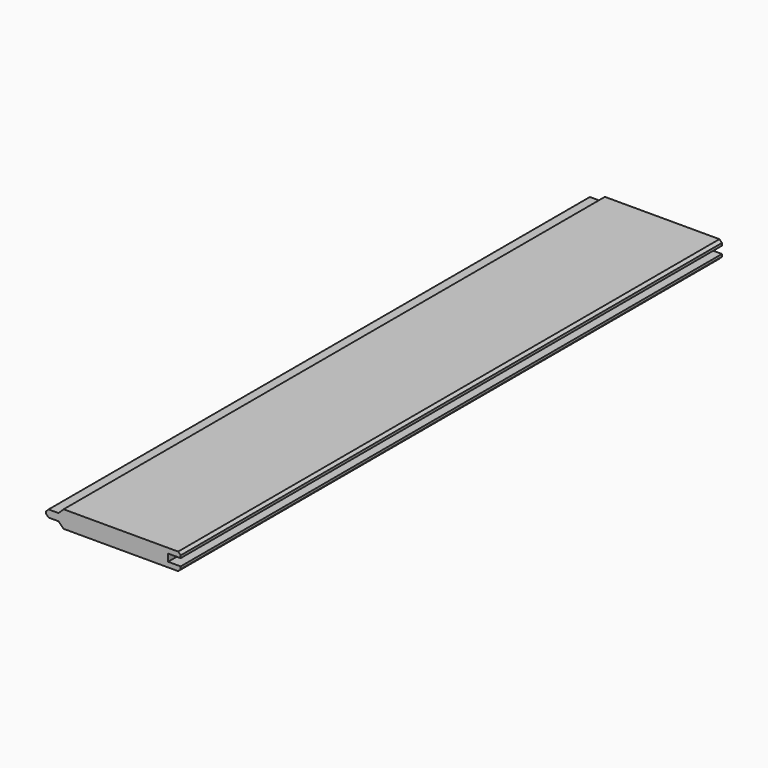
from build123d import *

# Parameters (mm, degrees)
F1_DEPTH = 685.8
F2_SIZE  = 2.54
F3_SIZE  = 5.07999


# Not quite as in the source:
# - a fillet or chamfer is up to 0.001 mm smaller than in the source, because OpenCascade refuses the exact size


with BuildPart() as f1:
    # F0 (on Front) → F1 (new body)
    with BuildSketch(Plane.XZ):
        Polygon((68.199, 3.6576), (68.199, 8.7376), (-55.499, 8.7376), (-55.499, 3.6576), (-68.199, 3.6576), (-68.199, -3.6576), (-55.499, -3.6576), (-55.499, -8.7376), (68.199, -8.7376), (68.199, -3.6576), (55.499, -3.6576), (55.499, 3.6576), align=None)
    extrude(amount=F1_DEPTH)

    # F2
    f2_edges = [f1.edges().sort_by_distance(p)[0] for p in [
        (68.199, -342.9, 8.7376),
        (68.199, -342.9, -8.7376),
        (-68.199, -342.9, 3.6576),
        (-68.199, -342.9, -3.6576),
    ]]
    chamfer(f2_edges, length=F2_SIZE)

    # F3 (size 5.08 in the source; OpenCascade refuses exactly that, so slightly less here)
    f3_edges = [f1.edges().sort_by_distance(p)[0] for p in [
        (-55.499, -342.9, 8.7376),
        (-55.499, -342.9, -8.7376),
    ]]
    chamfer(f3_edges, length=F3_SIZE)


solid = f1.part
